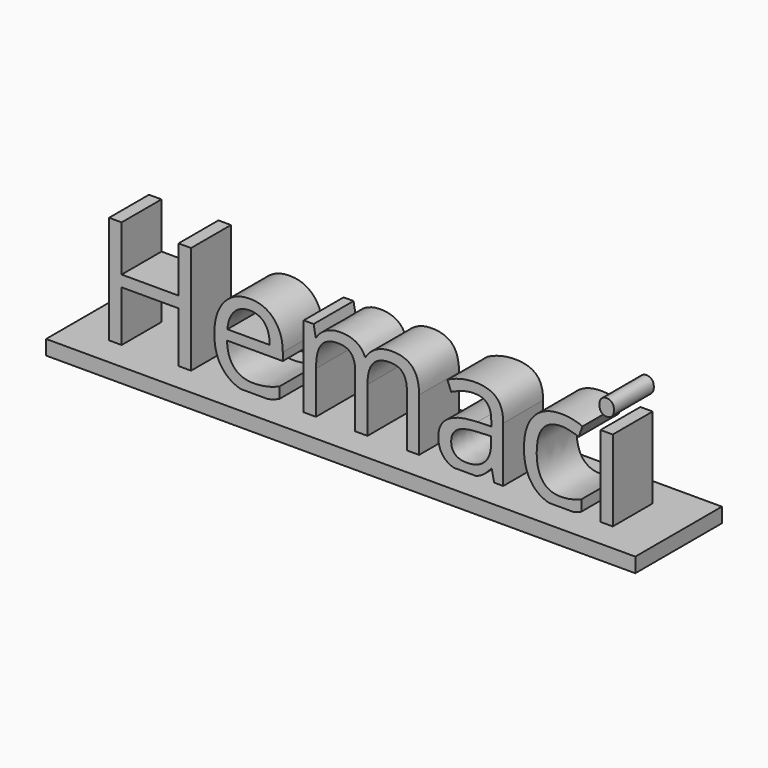
from build123d import *

# Parameters (mm, degrees)
F0_TEXT_SIZE = 39.3115786008
F1_DEPTH     = 12.954
F2_W         = 153.1479805708
F2_H         = 28.1425788999
F3_DEPTH     = 3.81


# Not quite as in the source:
# - Text() gives the source's letters only with a copy of the font that has no kerning and outlines rounded to 1/6400 em; it was checked with that copy


with BuildPart() as f1:
    # F0 (on Front) → F1 (new body)
    with BuildSketch(Plane.XZ):
        with Locations((-76.9012272358, 0)):
            Text('Hemaci', F0_TEXT_SIZE, font='Open Sans', text_align=(TextAlign.LEFT, TextAlign.BOTTOM))
    extrude(amount=F1_DEPTH)


with BuildPart() as f3:
    # F2 (on Top) → F3 (new body)
    with BuildSketch(Plane.XY):
        with Locations((-6.8486481905, -6.3793063164)):
            Rectangle(F2_W, F2_H)
    extrude(amount=-F3_DEPTH)


solid = Compound([f1.part, f3.part])
